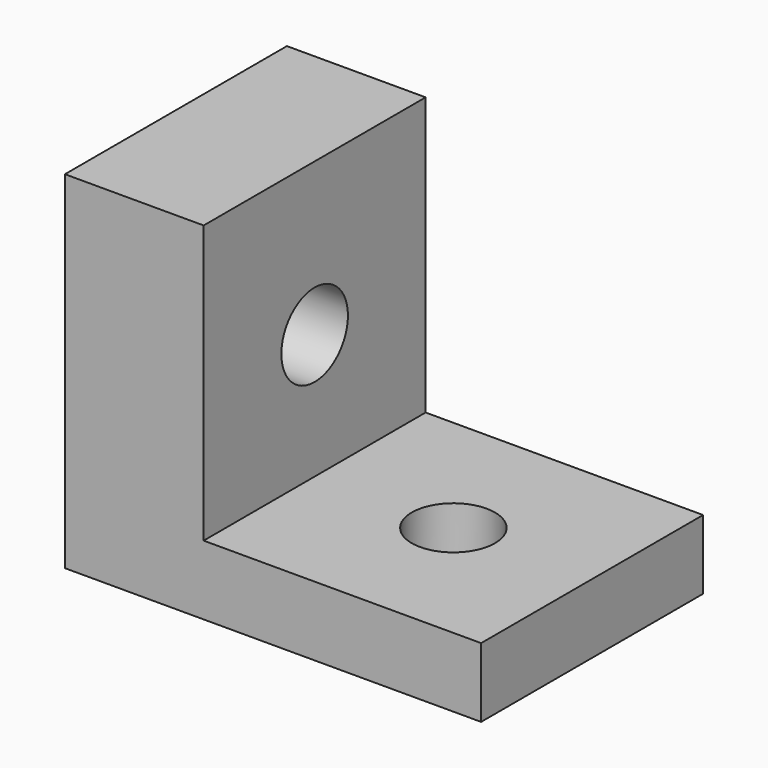
from build123d import *

# Parameters (mm, degrees)
F0_W     = 20
F0_H     = 20
F0_R     = 3
F1_DEPTH = 5
F0_W_2   = 10
F2_DEPTH = 25
F3_R     = 3
F4_DEPTH = 25


# Not quite as in the source:
# - a feature names something its author has since deleted; it is built from what else it names


with BuildPart() as f1:
    # F0 (on Top) → F1 (new body)
    with BuildSketch(Plane.XY):
        with Locations((20, 10)):
            Rectangle(F0_W, F0_H)
        with Locations((20, 10)):
            Circle(F0_R, mode=Mode.SUBTRACT)
    extrude(amount=F1_DEPTH)

    # F0 (on Top) → F2 (join)
    with BuildSketch(Plane.XY):
        with Locations((5, 10)):
            Rectangle(F0_W_2, F0_H)
    extrude(amount=F2_DEPTH)

    # F3 (on Right) → F4 (cut)
    with BuildSketch(Plane.YZ):
        with Locations((10, 14)):
            Circle(F3_R)
    extrude(amount=F4_DEPTH, mode=Mode.SUBTRACT)


solid = f1.part
